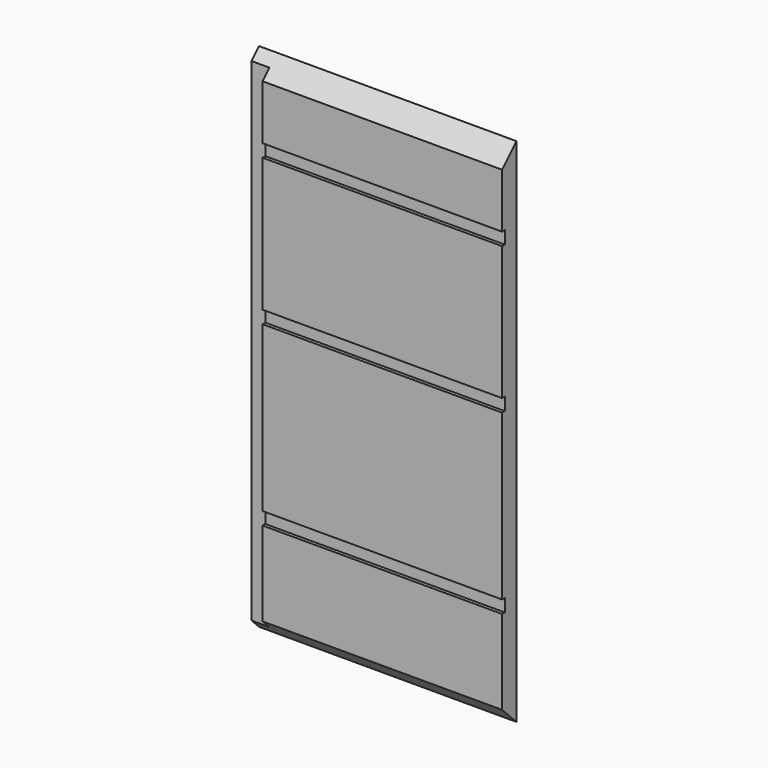
from build123d import *

# Parameters (mm, degrees)
F0_W     = 302
F0_H     = 600
F1_DEPTH = 21
F2_SIZE  = 20.99999
F3_W     = 21
F3_H     = 600
F4_DEPTH = 10
F5_W     = 302
F5_H     = 15
F6_DEPTH = 4
F7_W     = 281
F7_H     = 15
F8_DEPTH = 4


# Not quite as in the source:
# - a fillet or chamfer is up to 0.001 mm smaller than in the source, because OpenCascade refuses the exact size


with BuildPart() as f1:
    # F0 (on Front) → F1 (new body)
    with BuildSketch(Plane.XZ):
        with Locations((151, 300)):
            Rectangle(F0_W, F0_H)
    extrude(amount=-F1_DEPTH)

    # F2 (size 21 in the source; OpenCascade refuses exactly that, so slightly less here)
    f2_edges = [f1.edges().sort_by_distance(p)[0] for p in [
        (151, 0, 0),
        (151, 0, 600),
    ]]
    chamfer(f2_edges, length=F2_SIZE)

    # F3 (on face) → F4 (cut)
    with BuildSketch(Plane.XZ):
        with Locations((10.5, 300)):
            Rectangle(F3_W, F3_H)
    extrude(amount=-F4_DEPTH, mode=Mode.SUBTRACT)

    # F5 (on face) → F6 (cut)
    with BuildSketch(Plane.XZ):
        with Locations((151, 507.5)):
            Rectangle(F5_W, F5_H)
    extrude(amount=-F6_DEPTH, mode=Mode.SUBTRACT)

    # F7 (on face) → F8 (cut)
    with BuildSketch(Plane.XZ):
        with Locations((161.5, 335.5)):
            Rectangle(F7_W, F7_H)
        with Locations((161.5, 127.5)):
            Rectangle(F7_W, F7_H)
    extrude(amount=-F8_DEPTH, mode=Mode.SUBTRACT)


solid = f1.part
